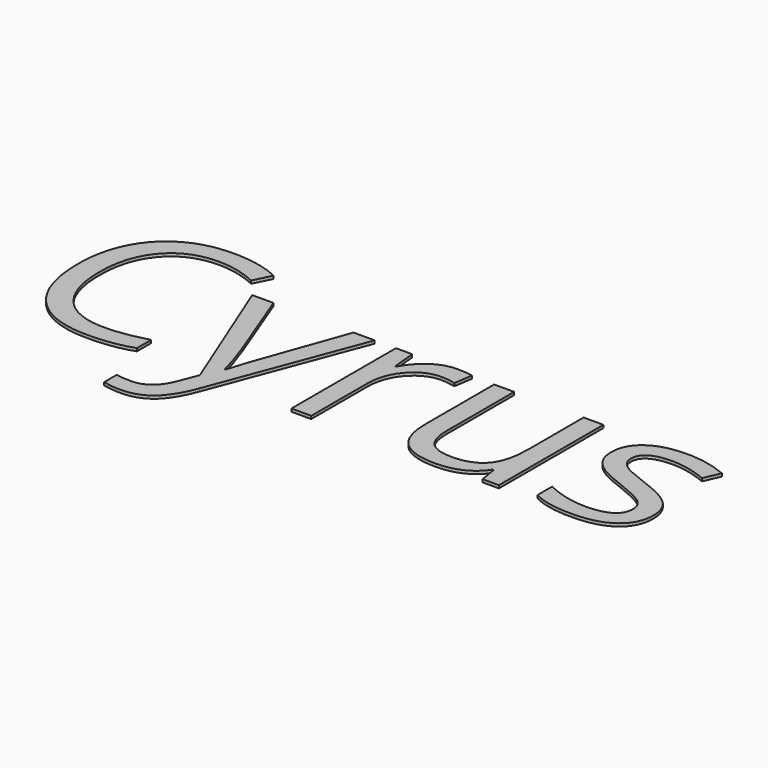
from build123d import *

# Parameters (mm, degrees)
F0_TEXT_SIZE = 211.3324590027
F1_DEPTH     = 2.54


# Not quite as in the source:
# - Text() gives the source's letters only with a copy of the font that has no kerning and outlines rounded to 1/6400 em; it was checked with that copy


with BuildPart() as f1:
    # F0 (on Top) → F1 (new body)
    with BuildSketch(Plane.XY):
        with Locations((-75.1672908664, -76.2902423739)):
            Text('Cyrus', F0_TEXT_SIZE, font='Open Sans', text_align=(TextAlign.LEFT, TextAlign.BOTTOM))
    extrude(amount=F1_DEPTH)


solid = f1.part
